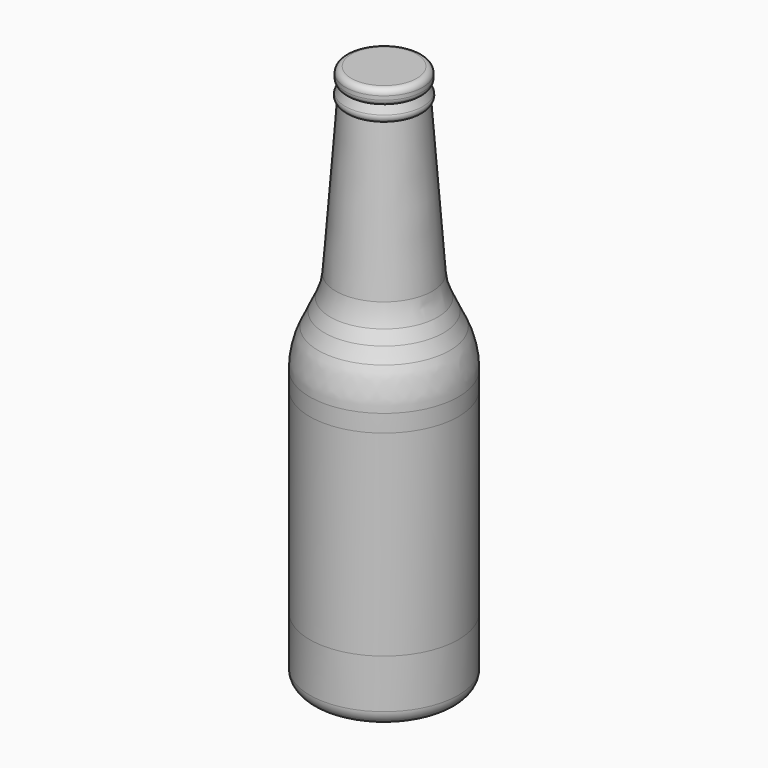
from build123d import *

# Parameters (mm, degrees)
F0_W   = 5
F0_H   = 21.4323662221
F0_W_2 = 12
F0_H_2 = 55
F0_H_3 = 5
F0_H_4 = 12.5676337779
F3_R   = 30
F4_R   = 20
F5_R   = 5
F0_H_5 = 66


# Not quite as in the source:
# - a fillet or chamfer that OpenCascade refuses, or shapes differently, is made with other operations: its cross-section is extruded or revolved along the edge and cut away or added


with BuildPart() as f1:
    # F0 (on Front) → F1 (revolve)
    with BuildSketch(Plane.XZ):
        with Locations((22.5, 10.7161831111)):
            Rectangle(F0_W, F0_H)
        Polygon((0, 118), (0, 0), (20, 0), (20, 21.4323662221), (20, 87.4323662221), (20, 100), (20, 110.5882352941), (16.5, 118), (12, 118), align=None)
        Polygon((20, 110.5882352941), (20, 100), (25, 100), align=None)
        Polygon((12, 173), (12, 118), (16.5, 118), (12.375, 173), align=None)
        with Locations((6, 145.5)):
            Rectangle(F0_W_2, F0_H_2)
        with Locations((6, 175.5)):
            Rectangle(F0_W_2, F0_H_3)
        Polygon((12, 178), (12, 173), (12.375, 173), align=None)
        Polygon((12, 178), (12.375, 173), (14, 173), align=None)
        Polygon((0, 183), (0, 178), (12, 178), (13, 178), (13, 183), align=None)
        with Locations((22.5, 93.7161831111)):
            Rectangle(F0_W, F0_H_4)
    revolve(axis=Axis((0, 0, 148), (0, 0, 1)))

    # F2: fillet of radius 2 on 3 edges, made by hand

    # F2_s1 → F2_t2 (revolve, cut)
    with BuildSketch(Plane.XZ):
        with BuildLine():
            ThreePointArc((13, 181), (12.4142135624, 182.4142135624), (11, 183))
            Line((11, 183), (11, 183.04))
            Line((11, 183.04), (13.04, 183.04))
            Line((13.04, 183.04), (13.04, 181))
            Line((13.04, 181), (13, 181))
        make_face()
    revolve(axis=Axis((0, 0, 183), (0, 0, 1)), mode=Mode.SUBTRACT)

    # F2_s3 → F2_t4 (revolve, cut)
    with BuildSketch(Plane.XZ):
        with BuildLine():
            ThreePointArc((12.375, 173), (13.1205394366, 174.0633553036), (13.055833561, 175.3604160974))
            Line((13.055833561, 175.3604160974), (13.0929726287, 175.3752717245))
            Line((13.0929726287, 175.3752717245), (14.0371390676, 173.0148556271))
            Line((14.0371390676, 173.0148556271), (14, 172.96))
            ThreePointArc((14, 172.96), (13.1875, 172.96), (12.3985223964, 172.9676473051))
            Line((12.3985223964, 172.9676473051), (12.375, 173))
        make_face()
    revolve(axis=Axis((0, 0, 173), (0, 0, 1)), mode=Mode.SUBTRACT)

    # F2_s5 → F2_t6 (revolve, cut)
    with BuildSketch(Plane.XZ):
        with BuildLine():
            ThreePointArc((12, 178), (12.7320508076, 178.7320508076), (13, 179.7320508076))
            Line((13, 179.7320508076), (13.04, 179.7320508076))
            Line((13.04, 179.7320508076), (13.04, 178))
            Line((13.04, 178), (13, 177.96))
            ThreePointArc((13, 177.96), (12.5, 177.96), (12.02, 177.9653589838))
            Line((12.02, 177.9653589838), (12, 178))
        make_face()
    revolve(axis=Axis((0, 0, 178), (0, 0, 1)), mode=Mode.SUBTRACT)

    # F3
    f3_edges = [f1.edges().sort_by_distance(p)[0] for p in [
        (-25, 0, 100),
    ]]
    fillet(f3_edges, radius=F3_R)

    # F4
    f4_edges = [f1.edges().sort_by_distance(p)[0] for p in [
        (-16.5, 0, 118),
    ]]
    fillet(f4_edges, radius=F4_R)

    # F5
    f5_edges = [f1.edges().sort_by_distance(p)[0] for p in [
        (-25, 0, 0),
    ]]
    fillet(f5_edges, radius=F5_R)

    # F6 (on Front) → F7 (revolve, cut)
    with BuildSketch(Plane.XZ):
        Polygon((0, 1.7939497484), (0, 0), (16.9230774045, 0), align=None)
    revolve(axis=Axis((0, 0, 0.8969748742), (0, 0, -1)), mode=Mode.SUBTRACT)


with BuildPart() as f8:
    # F0 (on Front) → F8 (revolve)
    with BuildSketch(Plane.XZ):
        with Locations((22.5, 54.4323662221)):
            Rectangle(F0_W, F0_H_5)
    revolve(axis=Axis((0, 0, 59), (0, 0, 1)))


solid = Compound([f1.part, f8.part])
